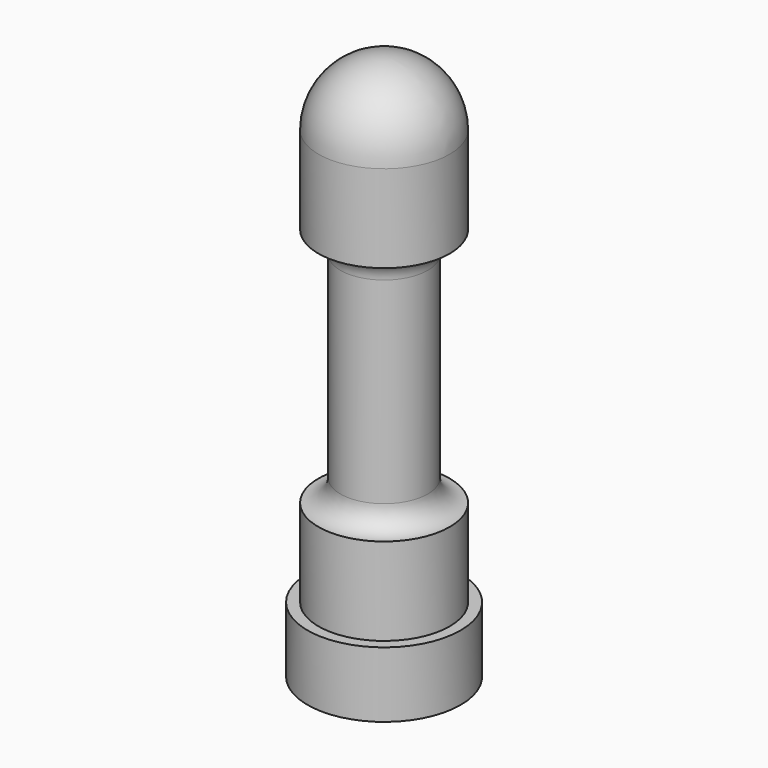
from build123d import *

# Parameters (mm, degrees)
F2_R = 0.99999


# Not quite as in the source:
# - a fillet or chamfer is up to 0.001 mm smaller than in the source, because OpenCascade refuses the exact size


with BuildPart() as f1:
    # F0 (on Front) → F1 (revolve)
    with BuildSketch(Plane.XZ):
        with BuildLine():
            Line((0, 25), (0, 22))
            Line((0, 22), (3, 22))
            ThreePointArc((3, 22), (2.1213203436, 24.1213203436), (0, 25))
        make_face()
        with BuildLine():
            ThreePointArc((0, 1.5), (1.0606601718, 1.0606601718), (1.5, 0))
            Line((1.5, 0), (3.5, 0))
            Line((3.5, 0), (3.5, 3))
            Line((3.5, 3), (3, 3))
            Line((3, 3), (3, 7))
            Line((3, 7), (2, 7))
            Line((2, 7), (2, 18))
            Line((2, 18), (3, 18))
            Line((3, 18), (3, 22))
            Line((3, 22), (0, 22))
            Line((0, 22), (0, 3))
            Line((0, 3), (0, 1.5))
        make_face()
    revolve(axis=Axis((0, 0, 13.25), (0, 0, -1)))

    # F2 (radius 1 in the source; OpenCascade refuses exactly that, so slightly less here)
    f2_edges = [f1.edges().sort_by_distance(p)[0] for p in [
        (-2, 0, 18),
        (-2, 0, 7),
    ]]
    fillet(f2_edges, radius=F2_R)


solid = f1.part
